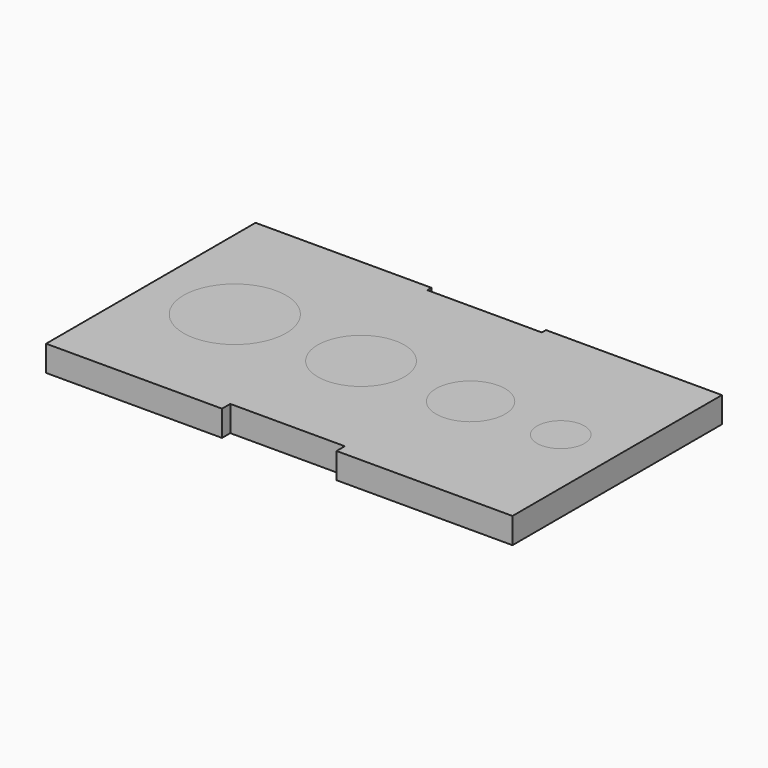
from build123d import *

# Parameters (mm, degrees)
F0_W   = 9.95
F0_H   = 5
F0_W_2 = 8.4
F0_W_3 = 6.7
F0_W_4 = 4.6


# Not quite as in the source:
# - a feature names something its author has since deleted; it is built from what else it names


with BuildPart() as f2:
    # F2: sweep along a path in F0
    with BuildLine(Plane.XZ) as f2_path:
        Line((-38.9, 0), (-38.9, 5))
    # F1 (on Top) → F2 (sweep)
    with BuildSketch(Plane.XY):
        Polygon((-11.1125, 25.4), (-45.25, 25.4), (-45.25, -25.4), (-11.1125, -25.4), (-11.1125, -23.4), (11.1125, -23.4), (11.1125, -25.4), (45.25, -25.4), (45.25, 25.4), (11.1125, 25.4), (11.1125, 24.4), (-11.1125, 24.4), align=None)
    sweep(path=f2_path.line)


with BuildPart() as f3:
    # F0 (on Front) → F3 (revolve)
    with BuildSketch(Plane.XZ):
        with Locations((-33.925, 2.5)):
            Rectangle(F0_W, F0_H)
    revolve(axis=Axis((-28.95, 0, 2.5), (0, 0, -1)))


with BuildPart() as f4:
    # F0 (on Front) → F4 (revolve)
    with BuildSketch(Plane.XZ):
        with Locations((-8.65, 2.5)):
            Rectangle(F0_W_2, F0_H)
    revolve(axis=Axis((-4.45, 0, 2.5), (0, 0, -1)))


with BuildPart() as f5:
    # F0 (on Front) → F5 (revolve)
    with BuildSketch(Plane.XZ):
        with Locations((13.45, 2.5)):
            Rectangle(F0_W_3, F0_H)
    revolve(axis=Axis((16.8, 0, 2.5), (0, 0, -1)))


with BuildPart() as f6:
    # F0 (on Front) → F6 (revolve)
    with BuildSketch(Plane.XZ):
        with Locations((32, 2.5)):
            Rectangle(F0_W_4, F0_H)
    revolve(axis=Axis((34.3, 0, 2.5), (0, 0, -1)))


with BuildPart() as f2_1:
    add(f2.part)

    # F7: cut F3, F4, F6, F5
    add(f3.part, mode=Mode.SUBTRACT)
    add(f4.part, mode=Mode.SUBTRACT)
    add(f6.part, mode=Mode.SUBTRACT)
    add(f5.part, mode=Mode.SUBTRACT)


solid = Compound([f3.part, f4.part, f5.part, f6.part, f2_1.part])
